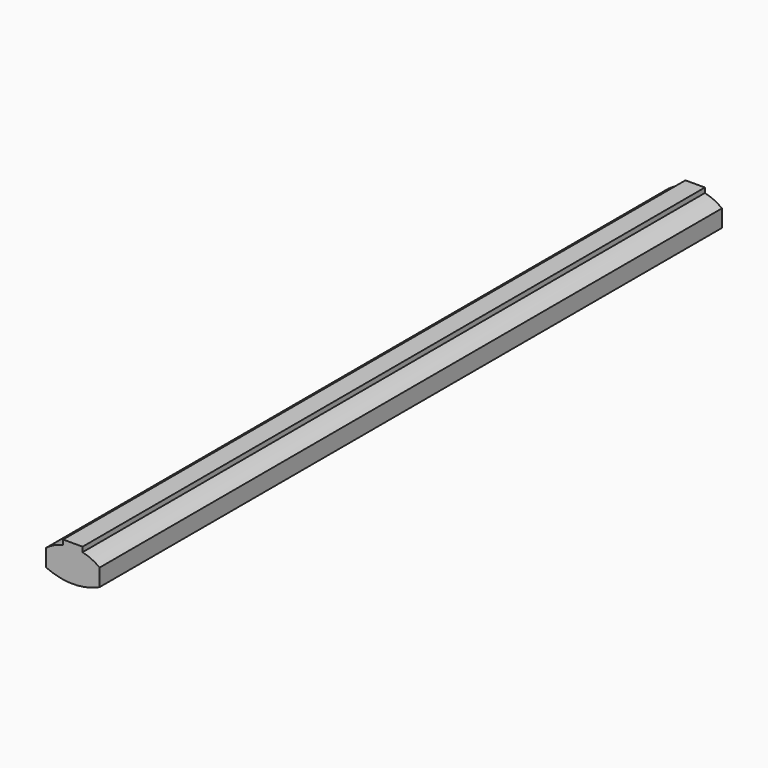
from build123d import *

# Parameters (mm, degrees)
F1_DEPTH = 1600


# Not quite as in the source:
# - ends of sketch curves that miss each other by under 0.0002 mm in the source are joined


with BuildPart() as f1:
    # F0 (on Front) → F1 (new body)
    with BuildSketch(Plane.XZ):
        with BuildLine():
            Line((54.9999419978, -17.7153473352), (55.0000580024, 17.7152582231))
            ThreePointArc((55.0000580024, 17.7152582231), (38.3907297006, 27.832811217), (20, 34.1586096885))
            Line((20, 34.1586096885), (20, 44.1586096885))
            Line((20, 44.1586096885), (-20, 44.1586096885))
            Line((-20, 44.1586096885), (-20, 34.1586096885))
            ThreePointArc((-20, 34.1586096885), (-38.390663502, 27.8328423177), (-54.9999419978, 17.7153473352))
            Line((-54.9999419978, 17.7153473352), (-55.0000580024, -17.7152582231))
            ThreePointArc((-55.0000580024, -17.7152582231), (-6.78258e-05, -29.8413903114), (54.9999419978, -17.7153473352))
        make_face()
    extrude(amount=F1_DEPTH)


solid = f1.part
